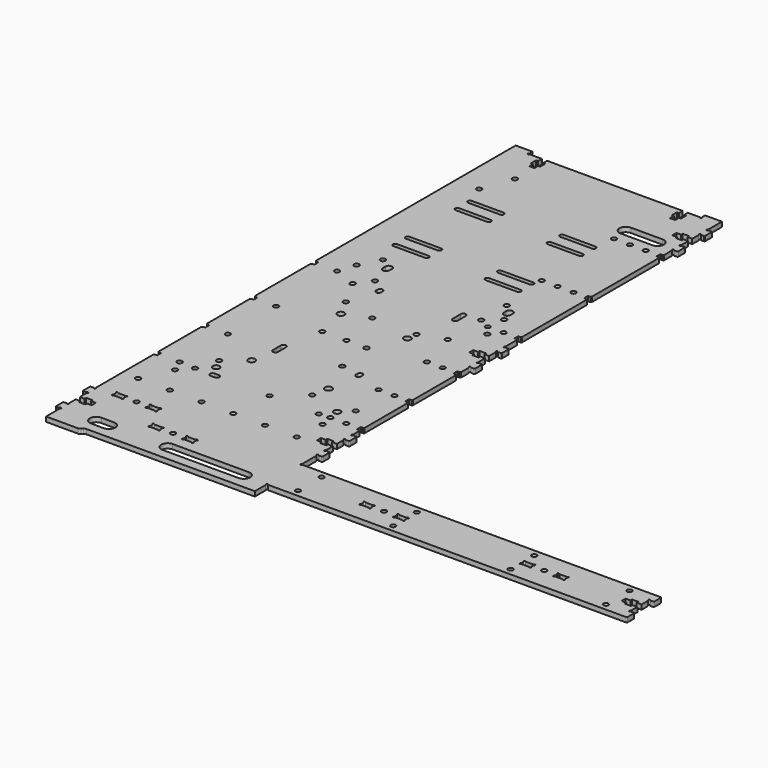
from build123d import *

# Parameters (mm, degrees)
F0_R     = 1.6
F0_R_2   = 1.55
F0_R_3   = 2.1
F0_R_4   = 2.225
F1_DEPTH = 3


# Not quite as in the source:
# - ends of sketch curves that miss each other by under 0.0002 mm in the source are joined


with BuildPart() as f1:
    # F0 (on Top) → F1 (new body)
    with BuildSketch(Plane.XY):
        with BuildLine():
            Line((-47.000029, -179.152731), (-47.000032, -170.618767))
            ThreePointArc((-47.000032, -170.618767), (-47.0670190274, -170.368768469), (-47.2500301961, -170.1857563396))
            ThreePointArc((-47.2500301961, -170.1857563396), (-47.3535809076, -169.3991911264), (-46.5670159066, -169.5027439461))
            ThreePointArc((-46.5670159066, -169.5027439461), (-46.3840030645, -169.6857566646), (-46.134003, -169.752744))
            Line((-46.134003, -169.752744), (179.500054, -169.752747))
            ThreePointArc((179.500054, -169.752747), (179.8536073906, -169.6063003906), (180.000054, -169.252747))
            Line((180.000054, -169.252747), (180.000054, -164.252749))
            ThreePointArc((180.000054, -164.252749), (179.8536073906, -163.8991956094), (179.500054, -163.752749))
            Line((179.500054, -163.752749), (177.866026, -163.752749))
            ThreePointArc((177.866026, -163.752749), (177.616026527, -163.8197359939), (177.4330139066, -164.0027479461))
            ThreePointArc((177.4330139066, -164.0027479461), (176.6464481264, -164.1062999076), (176.7500021291, -163.3197342236))
            ThreePointArc((176.7500021291, -163.3197342236), (176.9330146646, -163.1367210645), (177.000002, -162.886721))
            Line((177.000002, -162.886721), (177.000002, -157.752727))
            Line((177.000002, -157.752727), (174.00003, -157.752727))
            Line((174.00003, -157.752727), (174.00003, -159.027722))
            Line((174.00003, -159.027722), (170.000002, -159.027722))
            Line((170.000002, -159.027722), (170.000002, -157.752727))
            Line((170.000002, -157.752727), (167.000002, -157.752727))
            Line((167.000002, -157.752727), (167.000002, -154.552716))
            Line((167.000002, -154.552716), (170.000002, -154.552716))
            Line((170.000002, -154.552716), (170.000002, -153.277722))
            Line((170.000002, -153.277722), (174.00003, -153.277722))
            Line((174.00003, -153.277722), (174.00003, -154.552716))
            Line((174.00003, -154.552716), (177.000002, -154.552716))
            Line((177.000002, -154.552716), (176.999999, -149.418751))
            ThreePointArc((176.999999, -149.418751), (176.9330122226, -149.168751902), (176.7500008039, -148.9857393396))
            ThreePointArc((176.7500008039, -148.9857393396), (176.6464500924, -148.1991741264), (177.4330150934, -148.3027269461))
            ThreePointArc((177.4330150934, -148.3027269461), (177.6160279355, -148.4857396646), (177.866028, -148.552727))
            Line((177.866028, -148.552727), (179.500054, -148.55273))
            ThreePointArc((179.500054, -148.55273), (179.8536073906, -148.4062833906), (180.000054, -148.05273))
            Line((180.000054, -148.05273), (180.000054, -143.052733))
            ThreePointArc((180.000054, -143.052733), (179.8536073906, -142.6991796094), (179.500054, -142.552733))
            Line((179.500054, -142.552733), (-46.134005, -142.552733))
            ThreePointArc((-46.134005, -142.552733), (-46.384004098, -142.6197197774), (-46.5670166604, -142.8027311961))
            ThreePointArc((-46.5670166604, -142.8027311961), (-47.3535825674, -142.9062842138), (-47.2500288709, -142.1197182236))
            ThreePointArc((-47.2500288709, -142.1197182236), (-47.0670163354, -141.9367050645), (-47.000029, -141.686705))
            Line((-47.000029, -141.686705), (-47.000032, -130.618767))
            ThreePointArc((-47.000032, -130.618767), (-47.0670190274, -130.368768469), (-47.2500301961, -130.1857563396))
            ThreePointArc((-47.2500301961, -130.1857563396), (-47.3535809076, -129.3991911264), (-46.5670159066, -129.5027439461))
            ThreePointArc((-46.5670159066, -129.5027439461), (-46.3840030645, -129.6857566646), (-46.134003, -129.752744))
            Line((-46.134003, -129.752744), (-44.499977, -129.752747))
            ThreePointArc((-44.499977, -129.752747), (-44.1464236094, -129.6063003906), (-43.999977, -129.252747))
            Line((-43.999977, -129.252747), (-43.999977, -124.252749))
            ThreePointArc((-43.999977, -124.252749), (-44.1464236094, -123.8991956094), (-44.499977, -123.752749))
            Line((-44.499977, -123.752749), (-46.134005, -123.752749))
            ThreePointArc((-46.134005, -123.752749), (-46.384004098, -123.8197357774), (-46.5670166604, -124.0027471961))
            ThreePointArc((-46.5670166604, -124.0027471961), (-47.3535825674, -124.1063002138), (-47.2500288709, -123.3197342236))
            ThreePointArc((-47.2500288709, -123.3197342236), (-47.0670163354, -123.1367210645), (-47.000029, -122.886721))
            Line((-47.000029, -122.886721), (-47.000029, -117.752727))
            Line((-47.000029, -117.752727), (-50.000001, -117.752727))
            Line((-50.000001, -117.752727), (-50.000001, -119.027722))
            Line((-50.000001, -119.027722), (-54.000029, -119.027722))
            Line((-54.000029, -119.027722), (-54.000029, -117.752727))
            Line((-54.000029, -117.752727), (-57.000029, -117.752727))
            Line((-57.000029, -117.752727), (-57.000029, -114.552716))
            Line((-57.000029, -114.552716), (-54.000029, -114.552716))
            Line((-54.000029, -114.552716), (-54.000029, -113.277722))
            Line((-54.000029, -113.277722), (-50.000001, -113.277722))
            Line((-50.000001, -113.277722), (-50.000001, -114.552716))
            Line((-50.000001, -114.552716), (-47.000029, -114.552716))
            Line((-47.000029, -114.552716), (-47.000032, -109.418751))
            ThreePointArc((-47.000032, -109.418751), (-47.0670187774, -109.168751902), (-47.2500301961, -108.9857393396))
            ThreePointArc((-47.2500301961, -108.9857393396), (-47.3535809076, -108.1991741264), (-46.5670159066, -108.3027269461))
            ThreePointArc((-46.5670159066, -108.3027269461), (-46.3840030645, -108.4857396646), (-46.134003, -108.552727))
            Line((-46.134003, -108.552727), (-44.499977, -108.55273))
            ThreePointArc((-44.499977, -108.55273), (-44.1464236094, -108.4062833906), (-43.999977, -108.05273))
            Line((-43.999977, -108.05273), (-43.999977, -103.052733))
            ThreePointArc((-43.999977, -103.052733), (-44.1464236094, -102.6991796094), (-44.499977, -102.552733))
            Line((-44.499977, -102.552733), (-46.134005, -102.552733))
            ThreePointArc((-46.134005, -102.552733), (-46.384004098, -102.6197197774), (-46.5670166604, -102.8027311961))
            ThreePointArc((-46.5670166604, -102.8027311961), (-47.3535825674, -102.9062842138), (-47.2500288709, -102.1197182236))
            ThreePointArc((-47.2500288709, -102.1197182236), (-47.0670163354, -101.9367050645), (-47.000029, -101.686705))
            Line((-47.000029, -101.686705), (-47.000002, -96.652731))
            Line((-47.000002, -96.652731), (-47.499999, -96.152731))
            Line((-47.499999, -96.152731), (-48.999999, -96.152731))
            Line((-48.999999, -96.152731), (-48.999999, -93.152731))
            Line((-48.999999, -93.152731), (-47.499999, -93.152731))
            Line((-47.499999, -93.152731), (-46.999999, -92.652731))
            Line((-46.999999, -92.652731), (-46.999999, -58.652731))
            Line((-46.999999, -58.652731), (-47.499999, -58.152731))
            Line((-47.499999, -58.152731), (-48.999999, -58.152731))
            Line((-48.999999, -58.152731), (-48.999999, -55.152731))
            Line((-48.999999, -55.152731), (-47.499999, -55.152731))
            Line((-47.499999, -55.152731), (-46.999999, -54.652731))
            Line((-46.999999, -54.652731), (-46.999999, -20.652731))
            Line((-46.999999, -20.652731), (-47.499999, -20.152731))
            Line((-47.499999, -20.152731), (-48.999999, -20.152731))
            Line((-48.999999, -20.152731), (-48.999999, -17.152731))
            Line((-48.999999, -17.152731), (-47.499999, -17.152731))
            Line((-47.499999, -17.152731), (-47.000002, -16.652731))
            Line((-47.000002, -16.652731), (-47.000032, -10.618763))
            ThreePointArc((-47.000032, -10.618763), (-47.0670190274, -10.368764469), (-47.2500301961, -10.1857523396))
            ThreePointArc((-47.2500301961, -10.1857523396), (-47.3535809076, -9.3991871264), (-46.5670159066, -9.5027399461))
            ThreePointArc((-46.5670159066, -9.5027399461), (-46.3840030645, -9.6857526646), (-46.134003, -9.75274))
            Line((-46.134003, -9.75274), (-44.499977, -9.752743))
            ThreePointArc((-44.499977, -9.752743), (-44.1464236094, -9.6062963906), (-43.999977, -9.252743))
            Line((-43.999977, -9.252743), (-43.999977, -4.252745))
            ThreePointArc((-43.999977, -4.252745), (-44.1464236094, -3.8991916094), (-44.499977, -3.752745))
            Line((-44.499977, -3.752745), (-46.134005, -3.752745))
            ThreePointArc((-46.134005, -3.752745), (-46.384004098, -3.8197317774), (-46.5670166604, -4.0027431961))
            ThreePointArc((-46.5670166604, -4.0027431961), (-47.3535825674, -4.1062962138), (-47.2500288709, -3.3197302236))
            ThreePointArc((-47.2500288709, -3.3197302236), (-47.0670163354, -3.1367170645), (-47.000029, -2.886717))
            Line((-47.000029, -2.886717), (-47.000029, 2.247277))
            Line((-47.000029, 2.247277), (-50.000001, 2.247277))
            Line((-50.000001, 2.247277), (-50.000001, 0.972282))
            Line((-50.000001, 0.972282), (-54.000029, 0.972282))
            Line((-54.000029, 0.972282), (-54.000029, 2.247277))
            Line((-54.000029, 2.247277), (-57.000029, 2.247277))
            Line((-57.000029, 2.247277), (-57.000029, 5.447288))
            Line((-57.000029, 5.447288), (-54.000029, 5.447288))
            Line((-54.000029, 5.447288), (-54.000029, 6.722282))
            Line((-54.000029, 6.722282), (-50.000001, 6.722282))
            Line((-50.000001, 6.722282), (-50.000001, 5.447288))
            Line((-50.000001, 5.447288), (-47.000029, 5.447288))
            Line((-47.000029, 5.447288), (-47.000032, 10.581253))
            ThreePointArc((-47.000032, 10.581253), (-47.0670190274, 10.831251531), (-47.2500301961, 11.0142636604))
            ThreePointArc((-47.2500301961, 11.0142636604), (-47.3535809076, 11.8008288736), (-46.5670159066, 11.6972760539))
            ThreePointArc((-46.5670159066, 11.6972760539), (-46.3840030645, 11.5142633354), (-46.134003, 11.447276))
            Line((-46.134003, 11.447276), (-44.499977, 11.447273))
            ThreePointArc((-44.499977, 11.447273), (-44.1464236094, 11.5937196094), (-43.999977, 11.947273))
            Line((-43.999977, 11.947273), (-43.999977, 16.947271))
            ThreePointArc((-43.999977, 16.947271), (-44.1464236094, 17.3008243906), (-44.499977, 17.447271))
            Line((-44.499977, 17.447271), (-46.134005, 17.447271))
            ThreePointArc((-46.134005, 17.447271), (-46.384004098, 17.3802842226), (-46.5670166604, 17.1972728039))
            ThreePointArc((-46.5670166604, 17.1972728039), (-47.3535825674, 17.0937197862), (-47.2500288709, 17.8802857764))
            ThreePointArc((-47.2500288709, 17.8802857764), (-47.0670163354, 18.0632989355), (-47.000029, 18.313299))
            Line((-47.000029, 18.313299), (-47.000001, 27.347269))
            Line((-47.000001, 27.347269), (-47.499999, 27.847269))
            Line((-47.499999, 27.847269), (-48.999999, 27.847269))
            Line((-48.999999, 27.847269), (-48.999999, 30.847269))
            Line((-48.999999, 30.847269), (-47.499999, 30.847269))
            Line((-47.499999, 30.847269), (-46.999999, 31.347269))
            Line((-46.999999, 31.347269), (-46.999999, 82.347269))
            Line((-46.999999, 82.347269), (-47.499999, 82.847269))
            Line((-47.499999, 82.847269), (-48.999999, 82.847269))
            Line((-48.999999, 82.847269), (-48.999999, 85.847269))
            Line((-48.999999, 85.847269), (-47.499999, 85.847269))
            Line((-47.499999, 85.847269), (-46.999999, 86.347269))
            Line((-46.999999, 86.347269), (-46.999999, 139.347269))
            Line((-46.999999, 139.347269), (-47.499999, 139.847269))
            Line((-47.499999, 139.847269), (-48.999999, 139.847269))
            Line((-48.999999, 139.847269), (-48.999999, 142.847269))
            Line((-48.999999, 142.847269), (-47.499999, 142.847269))
            Line((-47.499999, 142.847269), (-47.000002, 143.347269))
            Line((-47.000002, 143.347269), (-47.000032, 149.381233))
            ThreePointArc((-47.000032, 149.381233), (-47.0670187774, 149.631232098), (-47.2500301961, 149.8142446604))
            ThreePointArc((-47.2500301961, 149.8142446604), (-47.3535809076, 150.6008098736), (-46.5670159066, 150.4972570539))
            ThreePointArc((-46.5670159066, 150.4972570539), (-46.3840030645, 150.3142443354), (-46.134003, 150.247257))
            Line((-46.134003, 150.247257), (-44.499977, 150.247254))
            ThreePointArc((-44.499977, 150.247254), (-44.1464236094, 150.3937006094), (-43.999977, 150.747254))
            Line((-43.999977, 150.747254), (-43.999977, 155.747251))
            ThreePointArc((-43.999977, 155.747251), (-44.1464236094, 156.1008043906), (-44.499977, 156.247251))
            Line((-44.499977, 156.247251), (-46.134005, 156.247251))
            ThreePointArc((-46.134005, 156.247251), (-46.384004098, 156.1802642226), (-46.5670166604, 155.9972528039))
            ThreePointArc((-46.5670166604, 155.9972528039), (-47.3535825674, 155.8936997862), (-47.2500288709, 156.6802657764))
            ThreePointArc((-47.2500288709, 156.6802657764), (-47.0670163354, 156.8632789355), (-47.000029, 157.113279))
            Line((-47.000029, 157.113279), (-47.000029, 162.247273))
            Line((-47.000029, 162.247273), (-50.000001, 162.247273))
            Line((-50.000001, 162.247273), (-50.000001, 160.972279))
            Line((-50.000001, 160.972279), (-54.000029, 160.972279))
            Line((-54.000029, 160.972279), (-54.000029, 162.247273))
            Line((-54.000029, 162.247273), (-57.000029, 162.247273))
            Line((-57.000029, 162.247273), (-57.000029, 165.447284))
            Line((-57.000029, 165.447284), (-54.000029, 165.447284))
            Line((-54.000029, 165.447284), (-54.000029, 166.722279))
            Line((-54.000029, 166.722279), (-50.000001, 166.722279))
            Line((-50.000001, 166.722279), (-50.000001, 165.447284))
            Line((-50.000001, 165.447284), (-47.000029, 165.447284))
            Line((-47.000029, 165.447284), (-47.000032, 170.581249))
            ThreePointArc((-47.000032, 170.581249), (-47.0670187774, 170.831248098), (-47.2500301961, 171.0142606604))
            ThreePointArc((-47.2500301961, 171.0142606604), (-47.3535809076, 171.8008258736), (-46.5670159066, 171.6972730539))
            ThreePointArc((-46.5670159066, 171.6972730539), (-46.3840030645, 171.5142603354), (-46.134003, 171.447273))
            Line((-46.134003, 171.447273), (-44.499977, 171.44727))
            ThreePointArc((-44.499977, 171.44727), (-44.1464236094, 171.5937166094), (-43.999977, 171.94727))
            Line((-43.999977, 171.94727), (-43.999977, 176.947267))
            ThreePointArc((-43.999977, 176.947267), (-44.1464236094, 177.3008203906), (-44.499977, 177.447267))
            Line((-44.499977, 177.447267), (-46.134005, 177.447267))
            ThreePointArc((-46.134005, 177.447267), (-46.384004098, 177.3802802226), (-46.5670166604, 177.1972688039))
            ThreePointArc((-46.5670166604, 177.1972688039), (-47.3535818736, 177.0937180924), (-47.2500290539, 177.8802830934))
            ThreePointArc((-47.2500290539, 177.8802830934), (-47.0670163354, 178.0632959355), (-47.000029, 178.313296))
            Line((-47.000029, 178.313296), (-47.000029, 188.847296))
            Line((-47.000029, 188.847296), (-57.650028, 188.847296))
            Line((-57.650028, 188.847296), (-57.650028, 186.613249))
            ThreePointArc((-57.650028, 186.613249), (-57.5830407896, 186.363249152), (-57.4000283039, 186.1802364736))
            ThreePointArc((-57.4000283039, 186.1802364736), (-57.2964738203, 185.3936713986), (-58.0830396604, 185.4972221961))
            ThreePointArc((-58.0830396604, 185.4972221961), (-58.266052527, 185.6802340061), (-58.516052, 185.747221))
            Line((-58.516052, 185.747221), (-66.050023, 185.747224))
            Line((-66.050023, 185.747224), (-66.050023, 182.747252))
            Line((-66.050023, 182.747252), (-64.775028, 182.747252))
            Line((-64.775028, 182.747252), (-64.775028, 178.747224))
            Line((-64.775028, 178.747224), (-66.050023, 178.747224))
            Line((-66.050023, 178.747224), (-66.050023, 175.747224))
            Line((-66.050023, 175.747224), (-69.250034, 175.747224))
            Line((-69.250034, 175.747224), (-69.250034, 178.747224))
            Line((-69.250034, 178.747224), (-70.525028, 178.747224))
            Line((-70.525028, 178.747224), (-70.525028, 182.747252))
            Line((-70.525028, 182.747252), (-69.250034, 182.747252))
            Line((-69.250034, 182.747252), (-69.250034, 185.747224))
            Line((-69.250034, 185.747224), (-154.749991, 185.746908))
            Line((-154.749991, 185.746908), (-154.749991, 182.746955))
            Line((-154.749991, 182.746955), (-153.474997, 182.746955))
            Line((-153.474997, 182.746955), (-153.474997, 178.746927))
            Line((-153.474997, 178.746927), (-154.749991, 178.746927))
            Line((-154.749991, 178.746927), (-154.749991, 175.746927))
            Line((-154.749991, 175.746927), (-157.950002, 175.746927))
            Line((-157.950002, 175.746927), (-157.950002, 178.746927))
            Line((-157.950002, 178.746927), (-159.224997, 178.746927))
            Line((-159.224997, 178.746927), (-159.224997, 182.746955))
            Line((-159.224997, 182.746955), (-157.950002, 182.746955))
            Line((-157.950002, 182.746955), (-157.950002, 185.746927))
            Line((-157.950002, 185.746927), (-165.483973, 185.746924))
            ThreePointArc((-165.483973, 185.746924), (-165.733972473, 185.6799370061), (-165.9169850934, 185.4969250539))
            ThreePointArc((-165.9169850934, 185.4969250539), (-166.7035498736, 185.3933740924), (-166.5999970539, 186.1799390934))
            ThreePointArc((-166.5999970539, 186.1799390934), (-166.4169843354, 186.3629519355), (-166.349997, 186.612952))
            Line((-166.349997, 186.612952), (-166.349997, 188.846999))
            Line((-166.349997, 188.846999), (-176.999999, 188.846999))
            Line((-176.999999, 188.846999), (-176.999999, 31.847269))
            ThreePointArc((-176.999999, 31.847269), (-176.7071057812, 31.1401622188), (-175.999999, 30.847269))
            Line((-175.999999, 30.847269), (-174.999999, 30.847269))
            Line((-174.999999, 30.847269), (-174.999999, 27.847269))
            Line((-174.999999, 27.847269), (-175.999999, 27.847269))
            ThreePointArc((-175.999999, 27.847269), (-176.7071057812, 27.5543757812), (-176.999999, 26.847269))
            Line((-176.999999, 26.847269), (-176.999999, -16.152731))
            ThreePointArc((-176.999999, -16.152731), (-176.7071057812, -16.8598377812), (-175.999999, -17.152731))
            Line((-175.999999, -17.152731), (-174.999999, -17.152731))
            Line((-174.999999, -17.152731), (-174.999999, -20.152731))
            Line((-174.999999, -20.152731), (-175.999999, -20.152731))
            ThreePointArc((-175.999999, -20.152731), (-176.7071057812, -20.4456242188), (-176.999999, -21.152731))
            Line((-176.999999, -21.152731), (-176.999999, -54.152731))
            ThreePointArc((-176.999999, -54.152731), (-176.7071057812, -54.8598377812), (-175.999999, -55.152731))
            Line((-175.999999, -55.152731), (-174.999999, -55.152731))
            Line((-174.999999, -55.152731), (-174.999999, -58.152731))
            Line((-174.999999, -58.152731), (-175.999999, -58.152731))
            ThreePointArc((-175.999999, -58.152731), (-176.7071057812, -58.4456242188), (-176.999999, -59.152731))
            Line((-176.999999, -59.152731), (-176.999999, -92.152731))
            ThreePointArc((-176.999999, -92.152731), (-176.7071057812, -92.8598377812), (-175.999999, -93.152731))
            Line((-175.999999, -93.152731), (-174.999999, -93.152731))
            Line((-174.999999, -93.152731), (-174.999999, -96.152731))
            Line((-174.999999, -96.152731), (-175.999999, -96.152731))
            ThreePointArc((-175.999999, -96.152731), (-176.7071057812, -96.4456242188), (-176.999999, -97.152731))
            Line((-176.999999, -97.152731), (-177.000001, -141.686705))
            ThreePointArc((-177.000001, -141.686705), (-176.9330137896, -141.936704848), (-176.7500013039, -142.1197175264))
            ThreePointArc((-176.7500013039, -142.1197175264), (-176.6464456435, -142.9062834247), (-177.4330120934, -142.8027320539))
            ThreePointArc((-177.4330120934, -142.8027320539), (-177.616024527, -142.6197199939), (-177.866024, -142.552733))
            Line((-177.866024, -142.552733), (-179.500053, -142.552733))
            ThreePointArc((-179.500053, -142.552733), (-179.8536063906, -142.6991796094), (-180.000053, -143.052733))
            Line((-180.000053, -143.052733), (-180.000053, -148.05273))
            ThreePointArc((-180.000053, -148.05273), (-179.8536063906, -148.4062833906), (-179.500053, -148.55273))
            Line((-179.500053, -148.55273), (-177.866026, -148.552727))
            ThreePointArc((-177.866026, -148.552727), (-177.616026152, -148.4857397896), (-177.4330134736, -148.3027273039))
            ThreePointArc((-177.4330134736, -148.3027273039), (-176.6464483986, -148.1991728203), (-176.7499991961, -148.9857386604))
            ThreePointArc((-176.7499991961, -148.9857386604), (-176.9330110061, -149.168751527), (-176.999998, -149.418751))
            Line((-176.999998, -149.418751), (-177.000001, -154.552716))
            Line((-177.000001, -154.552716), (-174.000029, -154.552716))
            Line((-174.000029, -154.552716), (-174.000029, -153.277722))
            Line((-174.000029, -153.277722), (-170.000001, -153.277722))
            Line((-170.000001, -153.277722), (-170.000001, -154.552716))
            Line((-170.000001, -154.552716), (-167.000001, -154.552716))
            Line((-167.000001, -154.552716), (-167.000001, -157.752727))
            Line((-167.000001, -157.752727), (-170.000001, -157.752727))
            Line((-170.000001, -157.752727), (-170.000001, -159.027722))
            Line((-170.000001, -159.027722), (-174.000029, -159.027722))
            Line((-174.000029, -159.027722), (-174.000029, -157.752727))
            Line((-174.000029, -157.752727), (-177.000001, -157.752727))
            Line((-177.000001, -157.752727), (-177.000001, -162.886721))
            ThreePointArc((-177.000001, -162.886721), (-176.9330137896, -163.136720848), (-176.7500013039, -163.3197335264))
            ThreePointArc((-176.7500013039, -163.3197335264), (-176.6464456435, -164.1062994247), (-177.4330120934, -164.0027480539))
            ThreePointArc((-177.4330120934, -164.0027480539), (-177.616024527, -163.8197359939), (-177.866024, -163.752749))
            Line((-177.866024, -163.752749), (-179.500053, -163.752749))
            ThreePointArc((-179.500053, -163.752749), (-179.8536063906, -163.8991956094), (-180.000053, -164.252749))
            Line((-180.000053, -164.252749), (-180.000053, -169.252747))
            ThreePointArc((-180.000053, -169.252747), (-179.8536063906, -169.6063003906), (-179.500053, -169.752747))
            Line((-179.500053, -169.752747), (-177.866026, -169.752744))
            ThreePointArc((-177.866026, -169.752744), (-177.616026152, -169.6857567896), (-177.4330134736, -169.5027443039))
            ThreePointArc((-177.4330134736, -169.5027443039), (-176.6464475753, -169.3991886435), (-176.7499989461, -170.1857550934))
            ThreePointArc((-176.7499989461, -170.1857550934), (-176.9330110061, -170.368767527), (-176.999998, -170.618767))
            Line((-176.999998, -170.618767), (-176.999999, -181.152731))
            Line((-176.999999, -181.152731), (-156.828457, -181.152731))
            ThreePointArc((-156.828457, -181.152731), (-156.0630911152, -181.0004904709), (-155.4142449376, -180.5669460624))
            Line((-155.4142449376, -180.5669460624), (-154.585813, -179.738516))
            ThreePointArc((-154.585813, -179.738516), (-153.9371645907, -179.3050534338), (-153.172029, -179.1527310458))
            Line((-153.172029, -179.1527310458), (-47.000029, -179.152731))
        make_face()
        with BuildLine():
            Line((-147.000028, -173.152731), (-155.000029, -173.152731))
            ThreePointArc((-155.000029, -173.152731), (-159.000029, -169.152731), (-155.000029, -165.152731))
            Line((-155.000029, -165.152731), (-147.000028, -165.152731))
            ThreePointArc((-147.000028, -165.152731), (-143.000028, -169.152731), (-147.000028, -173.152731))
        make_face(mode=Mode.SUBTRACT)
        with BuildLine():
            Line((-160.366025, -142.802693), (-164.833975, -142.802693))
            ThreePointArc((-164.833975, -142.802693), (-165.083974473, -142.8696799939), (-165.2669870934, -143.0526919461))
            ThreePointArc((-165.2669870934, -143.0526919461), (-166.0535533565, -143.1562434247), (-165.9499976879, -142.3696775406))
            ThreePointArc((-165.9499976879, -142.3696775406), (-165.7669852104, -142.186664848), (-165.699998, -141.936665))
            Line((-165.699998, -141.936665), (-165.700001, -140.368797))
            ThreePointArc((-165.700001, -140.368797), (-165.7669879939, -140.118797527), (-165.9499999461, -139.9357849066))
            ThreePointArc((-165.9499999461, -139.9357849066), (-166.0535506014, -139.1492188203), (-165.2669852236, -139.2527731291))
            ThreePointArc((-165.2669852236, -139.2527731291), (-165.083972848, -139.4357857896), (-164.833973, -139.502773))
            Line((-164.833973, -139.502773), (-160.366023, -139.50277))
            ThreePointArc((-160.366023, -139.50277), (-160.116023902, -139.4357832226), (-159.9330113396, -139.2527718039))
            ThreePointArc((-159.9330113396, -139.2527718039), (-159.1464449497, -139.1492192691), (-159.2500003121, -139.9357854594))
            ThreePointArc((-159.2500003121, -139.9357854594), (-159.4330130396, -140.118798585), (-159.5, -140.368799))
            Line((-159.5, -140.368799), (-159.499997, -141.936669))
            ThreePointArc((-159.499997, -141.936669), (-159.4330100061, -142.186668473), (-159.2499980539, -142.3696810934))
            ThreePointArc((-159.2499980539, -142.3696810934), (-159.1464473986, -143.1562471797), (-159.9330127764, -143.0526928709))
            ThreePointArc((-159.9330127764, -143.0526928709), (-160.116025152, -142.8696802104), (-160.366025, -142.802693))
        make_face(mode=Mode.SUBTRACT)
        with Locations((-151.999999, -141.152731)):
            Circle(F0_R, mode=Mode.SUBTRACT)
        with BuildLine():
            Line((-139.166026, -142.802693), (-143.633975, -142.802693))
            ThreePointArc((-143.633975, -142.802693), (-143.883974473, -142.8696799939), (-144.0669870934, -143.0526919461))
            ThreePointArc((-144.0669870934, -143.0526919461), (-144.8535531797, -143.1562426014), (-144.7499988709, -142.3696772236))
            ThreePointArc((-144.7499988709, -142.3696772236), (-144.5669862104, -142.186664848), (-144.499999, -141.936665))
            Line((-144.499999, -141.936665), (-144.500002, -140.368797))
            ThreePointArc((-144.500002, -140.368797), (-144.5669889939, -140.118797527), (-144.7500009461, -139.9357849066))
            ThreePointArc((-144.7500009461, -139.9357849066), (-144.8535516014, -139.1492188203), (-144.0669862236, -139.2527731291))
            ThreePointArc((-144.0669862236, -139.2527731291), (-143.883973848, -139.4357857896), (-143.633974, -139.502773))
            Line((-143.633974, -139.502773), (-139.166024, -139.50277))
            ThreePointArc((-139.166024, -139.50277), (-138.916024527, -139.4357830061), (-138.7330119066, -139.2527710539))
            ThreePointArc((-138.7330119066, -139.2527710539), (-137.9464458203, -139.1492203986), (-138.0500001291, -139.9357857764))
            ThreePointArc((-138.0500001291, -139.9357857764), (-138.2330130396, -140.118798585), (-138.3, -140.368799))
            Line((-138.3, -140.368799), (-138.299997, -141.936669))
            ThreePointArc((-138.299997, -141.936669), (-138.2330100061, -142.186668473), (-138.0499980539, -142.3696810934))
            ThreePointArc((-138.0499980539, -142.3696810934), (-137.9464473986, -143.1562471797), (-138.7330127764, -143.0526928709))
            ThreePointArc((-138.7330127764, -143.0526928709), (-138.916025585, -142.8696799604), (-139.166026, -142.802693))
        make_face(mode=Mode.SUBTRACT)
        with BuildLine():
            Line((-125.36596, -157.802674), (-129.83391, -157.802674))
            ThreePointArc((-129.83391, -157.802674), (-130.083909098, -157.8696607774), (-130.2669216604, -158.0526721961))
            ThreePointArc((-130.2669216604, -158.0526721961), (-131.0534880503, -158.1562247309), (-130.9499326879, -157.3696585406))
            ThreePointArc((-130.9499326879, -157.3696585406), (-130.7669202104, -157.186645848), (-130.699933, -156.936646))
            Line((-130.699933, -156.936646), (-130.699936, -155.368778))
            ThreePointArc((-130.699936, -155.368778), (-130.7669229939, -155.118778527), (-130.9499349461, -154.9357659066))
            ThreePointArc((-130.9499349461, -154.9357659066), (-131.0534856014, -154.1491998203), (-130.2669202236, -154.2527541291))
            ThreePointArc((-130.2669202236, -154.2527541291), (-130.083907848, -154.4357667896), (-129.833908, -154.502754))
            Line((-129.833908, -154.502754), (-125.365958, -154.502751))
            ThreePointArc((-125.365958, -154.502751), (-125.115958527, -154.4357640061), (-124.9329459066, -154.2527520539))
            ThreePointArc((-124.9329459066, -154.2527520539), (-124.1463796435, -154.1492005753), (-124.2499353121, -154.9357664594))
            ThreePointArc((-124.2499353121, -154.9357664594), (-124.4329480396, -155.118779585), (-124.499935, -155.36878))
            Line((-124.499935, -155.36878), (-124.499932, -156.93665))
            ThreePointArc((-124.499932, -156.93665), (-124.4329452226, -157.186649098), (-124.2499338039, -157.3696616604))
            ThreePointArc((-124.2499338039, -157.3696616604), (-124.146381963, -158.1562267441), (-124.9329473434, -158.0526736209))
            ThreePointArc((-124.9329473434, -158.0526736209), (-125.1159605024, -157.8696615854), (-125.36596, -157.802674))
        make_face(mode=Mode.SUBTRACT)
        with Locations((-116.999934, -156.152712)):
            Circle(F0_R, mode=Mode.SUBTRACT)
        with BuildLine():
            Line((-104.165961, -157.802674), (-108.63391, -157.802674))
            ThreePointArc((-108.63391, -157.802674), (-108.883909098, -157.8696607774), (-109.0669216604, -158.0526721961))
            ThreePointArc((-109.0669216604, -158.0526721961), (-109.8534878736, -158.1562239076), (-109.7499338709, -157.3696582236))
            ThreePointArc((-109.7499338709, -157.3696582236), (-109.5669212104, -157.186645848), (-109.499934, -156.936646))
            Line((-109.499934, -156.936646), (-109.499937, -155.368778))
            ThreePointArc((-109.499937, -155.368778), (-109.5669239939, -155.118778527), (-109.7499359461, -154.9357659066))
            ThreePointArc((-109.7499359461, -154.9357659066), (-109.8534866014, -154.1491998203), (-109.0669212236, -154.2527541291))
            ThreePointArc((-109.0669212236, -154.2527541291), (-108.883908848, -154.4357667896), (-108.633909, -154.502754))
            Line((-108.633909, -154.502754), (-104.165959, -154.502751))
            ThreePointArc((-104.165959, -154.502751), (-103.915959527, -154.4357640061), (-103.7329469066, -154.2527520539))
            ThreePointArc((-103.7329469066, -154.2527520539), (-102.9463819497, -154.1492012691), (-103.0499353791, -154.9357663434))
            ThreePointArc((-103.0499353791, -154.9357663434), (-103.2329480396, -155.118779585), (-103.299935, -155.36878))
            Line((-103.299935, -155.36878), (-103.299932, -156.93665))
            ThreePointArc((-103.299932, -156.93665), (-103.2329452226, -157.186649098), (-103.0499338039, -157.3696616604))
            ThreePointArc((-103.0499338039, -157.3696616604), (-102.946381963, -158.1562267441), (-103.7329473434, -158.0526736209))
            ThreePointArc((-103.7329473434, -158.0526736209), (-103.9159609355, -157.8696613354), (-104.165961, -157.802674))
        make_face(mode=Mode.SUBTRACT)
        with Locations((-167.000029, -121.152731)):
            Circle(F0_R, mode=Mode.SUBTRACT)
        with Locations((-147.000029, -121.152731)):
            Circle(F0_R, mode=Mode.SUBTRACT)
        with Locations((-158.500029, -102.652731)):
            Circle(F0_R, mode=Mode.SUBTRACT)
        with Locations((-161.999999, -94.652731)):
            Circle(F0_R, mode=Mode.SUBTRACT)
        with Locations((-151.882472, -95.165293)):
            Circle(F0_R, mode=Mode.SUBTRACT)
        with BuildLine():
            Line((-140.882429, -93.565331), (-138.144429, -93.565331))
            ThreePointArc((-138.144429, -93.565331), (-136.544429, -95.165331), (-138.144429, -96.765331))
            Line((-138.144429, -96.765331), (-140.882429, -96.765331))
            ThreePointArc((-140.882429, -96.765331), (-142.482429, -95.165331), (-140.882429, -93.565331))
        make_face(mode=Mode.SUBTRACT)
        with Locations((-127.000029, -121.152731)):
            Circle(F0_R, mode=Mode.SUBTRACT)
        with Locations((-107.000029, -121.152731)):
            Circle(F0_R, mode=Mode.SUBTRACT)
        with Locations((-104.882472, -95.165293)):
            Circle(F0_R, mode=Mode.SUBTRACT)
        with BuildLine():
            Line((-110.000029, -165.152731), (-62.000029, -165.152731))
            ThreePointArc((-62.000029, -165.152731), (-58.000029, -169.152731), (-62.000029, -173.152731))
            Line((-62.000029, -173.152731), (-110.000029, -173.152731))
            ThreePointArc((-110.000029, -173.152731), (-114.000029, -169.152731), (-110.000029, -165.152731))
        make_face(mode=Mode.SUBTRACT)
        with Locations((-30.753126, -165.446001)):
            Circle(F0_R_2, mode=Mode.SUBTRACT)
        with Locations((-30.753126, -146.859476)):
            Circle(F0_R_2, mode=Mode.SUBTRACT)
        with Locations((-87.000029, -121.152731)):
            Circle(F0_R, mode=Mode.SUBTRACT)
        with Locations((-67.000029, -121.152731)):
            Circle(F0_R, mode=Mode.SUBTRACT)
        with Locations((-73.882472, -95.165293)):
            Circle(F0_R, mode=Mode.SUBTRACT)
        with Locations((-65.500029, -102.652731)):
            Circle(F0_R, mode=Mode.SUBTRACT)
        with Locations((-66.999999, -94.652731)):
            Circle(F0_R, mode=Mode.SUBTRACT)
        with Locations((-56.999999, -94.652731)):
            Circle(F0_R_2, mode=Mode.SUBTRACT)
        with Locations((-147.729999, -81.442731)):
            Circle(F0_R, mode=Mode.SUBTRACT)
        with Locations((-144.391544, -87.774639)):
            Circle(F0_R_3, mode=Mode.SUBTRACT)
        with Locations((-135.390029, -71.152731)):
            Circle(F0_R_4, mode=Mode.SUBTRACT)
        with Locations((-162.000029, -56.652731)):
            Circle(F0_R_2, mode=Mode.SUBTRACT)
        with BuildLine():
            Line((-130.869999, -49.742731), (-130.869999, -56.092731))
            ThreePointArc((-130.869999, -56.092731), (-132.469999, -57.692731), (-134.069999, -56.092731))
            Line((-134.069999, -56.092731), (-134.069999, -49.742731))
            ThreePointArc((-134.069999, -49.742731), (-132.469999, -48.142731), (-130.869999, -49.742731))
        make_face(mode=Mode.SUBTRACT)
        with Locations((-96.629999, -48.242731)):
            Circle(F0_R, mode=Mode.SUBTRACT)
        with Locations((-162.000029, -18.652731)):
            Circle(F0_R_2, mode=Mode.SUBTRACT)
        with Locations((-127.389999, -25.612731)):
            Circle(F0_R, mode=Mode.SUBTRACT)
        with Locations((-112.229999, -25.442731)):
            Circle(F0_R, mode=Mode.SUBTRACT)
        with Locations((-99.449999, -25.612731)):
            Circle(F0_R, mode=Mode.SUBTRACT)
        with Locations((-132.080029, -5.052731)):
            Circle(F0_R_4, mode=Mode.SUBTRACT)
        with Locations((-117.229999, 1.057269)):
            Circle(F0_R, mode=Mode.SUBTRACT)
        with Locations((-90.170029, -5.052731)):
            Circle(F0_R_4, mode=Mode.SUBTRACT)
        with Locations((-89.029999, -81.442731)):
            Circle(F0_R, mode=Mode.SUBTRACT)
        with Locations((-68.191544, -87.774639)):
            Circle(F0_R_3, mode=Mode.SUBTRACT)
        with Locations((-87.000029, -71.152731)):
            Circle(F0_R_4, mode=Mode.SUBTRACT)
        with Locations((-61.729999, -81.242731)):
            Circle(F0_R, mode=Mode.SUBTRACT)
        with BuildLine():
            Line((-82.609999, -49.742731), (-82.609999, -51.012731))
            ThreePointArc((-82.609999, -51.012731), (-84.209999, -52.612731), (-85.809999, -51.012731))
            Line((-85.809999, -51.012731), (-85.809999, -49.742731))
            ThreePointArc((-85.809999, -49.742731), (-84.209999, -48.142731), (-82.609999, -49.742731))
        make_face(mode=Mode.SUBTRACT)
        with Locations((-66.999999, -56.652731)):
            Circle(F0_R, mode=Mode.SUBTRACT)
        with Locations((-56.999999, -56.652731)):
            Circle(F0_R_2, mode=Mode.SUBTRACT)
        with Locations((-89.289999, 1.057269)):
            Circle(F0_R, mode=Mode.SUBTRACT)
        with Locations((-66.999999, -18.652731)):
            Circle(F0_R, mode=Mode.SUBTRACT)
        with Locations((-56.999999, -18.652731)):
            Circle(F0_R_2, mode=Mode.SUBTRACT)
        with Locations((29.246874, -165.446001)):
            Circle(F0_R_2, mode=Mode.SUBTRACT)
        with BuildLine():
            Line((7.633897, -157.802684), (3.165947, -157.802684))
            ThreePointArc((3.165947, -157.802684), (2.915947902, -157.8696707774), (2.7329353396, -158.0526821961))
            ThreePointArc((2.7329353396, -158.0526821961), (1.9463688203, -158.1562336014), (2.0499238791, -157.3696677906))
            ThreePointArc((2.0499238791, -157.3696677906), (2.2329366646, -157.1866550645), (2.299924, -156.936655))
            Line((2.299924, -156.936655), (2.299921, -155.368788))
            ThreePointArc((2.299921, -155.368788), (2.2329342226, -155.118788902), (2.0499228039, -154.9357763396))
            ThreePointArc((2.0499228039, -154.9357763396), (1.9463719156, -154.1492103032), (2.7329370934, -154.2527629461))
            ThreePointArc((2.7329370934, -154.2527629461), (2.9159495024, -154.4357764146), (3.165949, -154.502764))
            Line((3.165949, -154.502764), (7.633899, -154.502761))
            ThreePointArc((7.633899, -154.502761), (7.883898473, -154.4357740061), (8.0669110934, -154.2527620539))
            ThreePointArc((8.0669110934, -154.2527620539), (8.8534771797, -154.1492103986), (8.7499221209, -154.9357762094))
            ThreePointArc((8.7499221209, -154.9357762094), (8.5669090854, -155.1187893685), (8.499922, -155.36879))
            Line((8.499922, -155.36879), (8.499925, -156.936659))
            ThreePointArc((8.499925, -156.936659), (8.5669119939, -157.186658473), (8.7499239461, -157.3696710934))
            ThreePointArc((8.7499239461, -157.3696710934), (8.8534750844, -158.1562366968), (8.0669099066, -158.0526840539))
            ThreePointArc((8.0669099066, -158.0526840539), (7.8838970645, -157.8696713354), (7.633897, -157.802684))
        make_face(mode=Mode.SUBTRACT)
        with Locations((15.999923, -156.152721)):
            Circle(F0_R, mode=Mode.SUBTRACT)
        with BuildLine():
            Line((28.833896, -157.802684), (24.365947, -157.802684))
            ThreePointArc((24.365947, -157.802684), (24.115947902, -157.8696707774), (23.9329353396, -158.0526821961))
            ThreePointArc((23.9329353396, -158.0526821961), (23.1463701264, -158.1562329076), (23.2499229461, -157.3696679066))
            ThreePointArc((23.2499229461, -157.3696679066), (23.4329356646, -157.1866550645), (23.499923, -156.936655))
            Line((23.499923, -156.936655), (23.49992, -155.368788))
            ThreePointArc((23.49992, -155.368788), (23.4329332226, -155.118788902), (23.2499218039, -154.9357763396))
            ThreePointArc((23.2499218039, -154.9357763396), (23.1463709156, -154.1492103032), (23.9329360934, -154.2527629461))
            ThreePointArc((23.9329360934, -154.2527629461), (24.1159485024, -154.4357764146), (24.365948, -154.502764))
            Line((24.365948, -154.502764), (28.833898, -154.502761))
            ThreePointArc((28.833898, -154.502761), (29.083897473, -154.4357740061), (29.2669100934, -154.2527620539))
            ThreePointArc((29.2669100934, -154.2527620539), (30.053476003, -154.1492112218), (29.9499223039, -154.9357765264))
            ThreePointArc((29.9499223039, -154.9357765264), (29.7669090854, -155.1187893685), (29.699922, -155.36879))
            Line((29.699922, -155.36879), (29.699925, -156.936659))
            ThreePointArc((29.699925, -156.936659), (29.7669119939, -157.186658473), (29.9499239461, -157.3696710934))
            ThreePointArc((29.9499239461, -157.3696710934), (30.0534750844, -158.1562366968), (29.2669099066, -158.0526840539))
            ThreePointArc((29.2669099066, -158.0526840539), (29.0838962565, -157.8696708689), (28.833896, -157.802684))
        make_face(mode=Mode.SUBTRACT)
        with Locations((29.246874, -146.859476)):
            Circle(F0_R_2, mode=Mode.SUBTRACT)
        with Locations((103.246874, -165.446001)):
            Circle(F0_R_2, mode=Mode.SUBTRACT)
        with BuildLine():
            Line((108.634012, -157.802639), (104.166062, -157.802639))
            ThreePointArc((104.166062, -157.802639), (103.916062902, -157.8696257774), (103.7330503396, -158.0526371961))
            ThreePointArc((103.7330503396, -158.0526371961), (102.9464838203, -158.1561886014), (103.0500388791, -157.3696227906))
            ThreePointArc((103.0500388791, -157.3696227906), (103.2330516646, -157.1866100645), (103.300039, -156.93661))
            Line((103.300039, -156.93661), (103.300036, -155.368743))
            ThreePointArc((103.300036, -155.368743), (103.2330490061, -155.118743527), (103.0500370539, -154.9357309066))
            ThreePointArc((103.0500370539, -154.9357309066), (102.9464862218, -154.149164997), (103.7330515264, -154.2527186961))
            ThreePointArc((103.7330515264, -154.2527186961), (103.9160639355, -154.4357316646), (104.166064, -154.502719))
            Line((104.166064, -154.502719), (108.634014, -154.502716))
            ThreePointArc((108.634014, -154.502716), (108.8840132565, -154.4357291311), (109.0670258434, -154.2527174869))
            ThreePointArc((109.0670258434, -154.2527174869), (109.853592003, -154.1491652218), (109.7500371209, -154.9357312094))
            ThreePointArc((109.7500371209, -154.9357312094), (109.5670240854, -155.1187443685), (109.500037, -155.368745))
            Line((109.500037, -155.368745), (109.50004, -156.936615))
            ThreePointArc((109.50004, -156.936615), (109.5670267774, -157.186614098), (109.7500381961, -157.3696266604))
            ThreePointArc((109.7500381961, -157.3696266604), (109.8535889076, -158.1561918736), (109.0670239066, -158.0526390539))
            ThreePointArc((109.0670239066, -158.0526390539), (108.8840114976, -157.8696265854), (108.634012, -157.802639))
        make_face(mode=Mode.SUBTRACT)
        with Locations((103.246874, -146.859478)):
            Circle(F0_R_2, mode=Mode.SUBTRACT)
        with Locations((117.000038, -156.152677)):
            Circle(F0_R, mode=Mode.SUBTRACT)
        with BuildLine():
            Line((129.834011, -157.802639), (125.366062, -157.802639))
            ThreePointArc((125.366062, -157.802639), (125.116062902, -157.8696257774), (124.9330503396, -158.0526371961))
            ThreePointArc((124.9330503396, -158.0526371961), (124.146483997, -158.1561877782), (124.2500376961, -157.3696224736))
            ThreePointArc((124.2500376961, -157.3696224736), (124.4330506646, -157.1866100645), (124.500038, -156.93661))
            Line((124.500038, -156.93661), (124.500035, -155.368743))
            ThreePointArc((124.500035, -155.368743), (124.4330480061, -155.118743527), (124.2500360539, -154.9357309066))
            ThreePointArc((124.2500360539, -154.9357309066), (124.1464852218, -154.149164997), (124.9330505264, -154.2527186961))
            ThreePointArc((124.9330505264, -154.2527186961), (125.1160629355, -154.4357316646), (125.366063, -154.502719))
            Line((125.366063, -154.502719), (129.834013, -154.502716))
            ThreePointArc((129.834013, -154.502716), (130.0840122565, -154.4357291311), (130.2670248434, -154.2527174869))
            ThreePointArc((130.2670248434, -154.2527174869), (131.0535896968, -154.1491659156), (130.9500370539, -154.9357310934))
            ThreePointArc((130.9500370539, -154.9357310934), (130.7670240854, -155.1187443685), (130.700037, -155.368745))
            Line((130.700037, -155.368745), (130.70004, -156.936615))
            ThreePointArc((130.70004, -156.936615), (130.7670267774, -157.186614098), (130.9500381961, -157.3696266604))
            ThreePointArc((130.9500381961, -157.3696266604), (131.0535889076, -158.1561918736), (130.2670239066, -158.0526390539))
            ThreePointArc((130.2670239066, -158.0526390539), (130.0840110645, -157.8696263354), (129.834011, -157.802639))
        make_face(mode=Mode.SUBTRACT)
        with Locations((163.246874, -165.446001)):
            Circle(F0_R_2, mode=Mode.SUBTRACT)
        with Locations((163.247001, -146.859431)):
            Circle(F0_R_2, mode=Mode.SUBTRACT)
        with Locations((-138.144472, 6.434707)):
            Circle(F0_R, mode=Mode.SUBTRACT)
        with Locations((-147.729999, 23.757269)):
            Circle(F0_R, mode=Mode.SUBTRACT)
        with Locations((-162.000029, 29.347269)):
            Circle(F0_R_2, mode=Mode.SUBTRACT)
        with Locations((-158.500029, 40.347269)):
            Circle(F0_R, mode=Mode.SUBTRACT)
        with Locations((-140.882472, 32.834707)):
            Circle(F0_R, mode=Mode.SUBTRACT)
        with BuildLine():
            Line((-146.491544, 46.025361), (-146.491544, 48.025361))
            ThreePointArc((-146.491544, 48.025361), (-144.391544, 50.125361), (-142.291544, 48.025361))
            Line((-142.291544, 48.025361), (-142.291544, 46.025361))
            ThreePointArc((-142.291544, 46.025361), (-144.391544, 43.925361), (-146.491544, 46.025361))
        make_face(mode=Mode.SUBTRACT)
        with BuildLine():
            Line((-134.069999, 25.187269), (-134.069999, 26.457269))
            ThreePointArc((-134.069999, 26.457269), (-132.469999, 28.057269), (-130.869999, 26.457269))
            Line((-130.869999, 26.457269), (-130.869999, 25.187269))
            ThreePointArc((-130.869999, 25.187269), (-132.469999, 23.587269), (-134.069999, 25.187269))
        make_face(mode=Mode.SUBTRACT)
        with Locations((-151.882472, 52.834707)):
            Circle(F0_R, mode=Mode.SUBTRACT)
        with BuildLine():
            Line((-137.000029, 67.472269), (-157.000029, 67.472269))
            ThreePointArc((-157.000029, 67.472269), (-158.375029, 68.847269), (-157.000029, 70.222269))
            Line((-157.000029, 70.222269), (-137.000029, 70.222269))
            ThreePointArc((-137.000029, 70.222269), (-135.625029, 68.847269), (-137.000029, 67.472269))
        make_face(mode=Mode.SUBTRACT)
        with BuildLine():
            Line((-137.000029, 77.472269), (-157.000029, 77.472269))
            ThreePointArc((-157.000029, 77.472269), (-158.375029, 78.847269), (-157.000029, 80.222269))
            Line((-157.000029, 80.222269), (-137.000029, 80.222269))
            ThreePointArc((-137.000029, 80.222269), (-135.625029, 78.847269), (-137.000029, 77.472269))
        make_face(mode=Mode.SUBTRACT)
        with Locations((-73.882472, 6.434707)):
            Circle(F0_R, mode=Mode.SUBTRACT)
        with Locations((-62.229999, 23.057269)):
            Circle(F0_R, mode=Mode.SUBTRACT)
        with BuildLine():
            Line((-82.609999, 31.537269), (-82.609999, 25.187269))
            ThreePointArc((-82.609999, 25.187269), (-84.209999, 23.587269), (-85.809999, 25.187269))
            Line((-85.809999, 25.187269), (-85.809999, 31.537269))
            ThreePointArc((-85.809999, 31.537269), (-84.209999, 33.137269), (-82.609999, 31.537269))
        make_face(mode=Mode.SUBTRACT)
        with Locations((-73.882472, 32.834707)):
            Circle(F0_R, mode=Mode.SUBTRACT)
        with BuildLine():
            Line((-70.291544, 46.025361), (-70.291544, 48.025361))
            ThreePointArc((-70.291544, 48.025361), (-68.191544, 50.125361), (-66.091544, 48.025361))
            Line((-66.091544, 48.025361), (-66.091544, 46.025361))
            ThreePointArc((-66.091544, 46.025361), (-68.191544, 43.925361), (-70.291544, 46.025361))
        make_face(mode=Mode.SUBTRACT)
        with Locations((-66.999999, 29.347269)):
            Circle(F0_R_2, mode=Mode.SUBTRACT)
        with Locations((-56.999999, 29.347269)):
            Circle(F0_R_2, mode=Mode.SUBTRACT)
        with Locations((-65.500029, 40.347269)):
            Circle(F0_R, mode=Mode.SUBTRACT)
        with Locations((-73.882472, 52.834707)):
            Circle(F0_R, mode=Mode.SUBTRACT)
        with BuildLine():
            Line((-79.000029, 67.472269), (-99.000029, 67.472269))
            ThreePointArc((-99.000029, 67.472269), (-100.375029, 68.847269), (-99.000029, 70.222269))
            Line((-99.000029, 70.222269), (-79.000029, 70.222269))
            ThreePointArc((-79.000029, 70.222269), (-77.625029, 68.847269), (-79.000029, 67.472269))
        make_face(mode=Mode.SUBTRACT)
        with BuildLine():
            Line((-79.000029, 77.472269), (-99.000029, 77.472269))
            ThreePointArc((-99.000029, 77.472269), (-100.375029, 78.847269), (-99.000029, 80.222269))
            Line((-99.000029, 80.222269), (-79.000029, 80.222269))
            ThreePointArc((-79.000029, 80.222269), (-77.625029, 78.847269), (-79.000029, 77.472269))
        make_face(mode=Mode.SUBTRACT)
        with Locations((-76.999999, 84.347269)):
            Circle(F0_R_2, mode=Mode.SUBTRACT)
        with Locations((-66.999999, 84.347269)):
            Circle(F0_R_2, mode=Mode.SUBTRACT)
        with Locations((-56.999999, 84.347269)):
            Circle(F0_R_2, mode=Mode.SUBTRACT)
        with BuildLine():
            Line((-137.000029, 116.472269), (-157.000029, 116.472269))
            ThreePointArc((-157.000029, 116.472269), (-158.375029, 117.847269), (-157.000029, 119.222269))
            Line((-157.000029, 119.222269), (-137.000029, 119.222269))
            ThreePointArc((-137.000029, 119.222269), (-135.625029, 117.847269), (-137.000029, 116.472269))
        make_face(mode=Mode.SUBTRACT)
        with Locations((-161.999999, 141.347269)):
            Circle(F0_R_2, mode=Mode.SUBTRACT)
        with BuildLine():
            Line((-137.000029, 126.472269), (-157.000029, 126.472269))
            ThreePointArc((-157.000029, 126.472269), (-158.375029, 127.847269), (-157.000029, 129.222269))
            Line((-157.000029, 129.222269), (-137.000029, 129.222269))
            ThreePointArc((-137.000029, 129.222269), (-135.625029, 127.847269), (-137.000029, 126.472269))
        make_face(mode=Mode.SUBTRACT)
        with Locations((-154.999999, 160.747269)):
            Circle(F0_R, mode=Mode.SUBTRACT)
        with BuildLine():
            Line((-79.000029, 116.472269), (-99.000029, 116.472269))
            ThreePointArc((-99.000029, 116.472269), (-100.375029, 117.847269), (-99.000029, 119.222269))
            Line((-99.000029, 119.222269), (-79.000029, 119.222269))
            ThreePointArc((-79.000029, 119.222269), (-77.625029, 117.847269), (-79.000029, 116.472269))
        make_face(mode=Mode.SUBTRACT)
        with BuildLine():
            Line((-79.000029, 126.472269), (-99.000029, 126.472269))
            ThreePointArc((-99.000029, 126.472269), (-100.375029, 127.847269), (-99.000029, 129.222269))
            Line((-99.000029, 129.222269), (-79.000029, 129.222269))
            ThreePointArc((-79.000029, 129.222269), (-77.625029, 127.847269), (-79.000029, 126.472269))
        make_face(mode=Mode.SUBTRACT)
        with Locations((-76.999999, 141.347269)):
            Circle(F0_R_2, mode=Mode.SUBTRACT)
        with Locations((-66.999999, 141.347269)):
            Circle(F0_R_2, mode=Mode.SUBTRACT)
        with Locations((-56.999999, 141.347269)):
            Circle(F0_R_2, mode=Mode.SUBTRACT)
        with BuildLine():
            Line((-57.999999, 147.847269), (-77.999999, 147.847269))
            ThreePointArc((-77.999999, 147.847269), (-81.999999, 151.847269), (-77.999999, 155.847269))
            Line((-77.999999, 155.847269), (-57.999999, 155.847269))
            ThreePointArc((-57.999999, 155.847269), (-53.999999, 151.847269), (-57.999999, 147.847269))
        make_face(mode=Mode.SUBTRACT)
    extrude(amount=F1_DEPTH)


solid = f1.part
